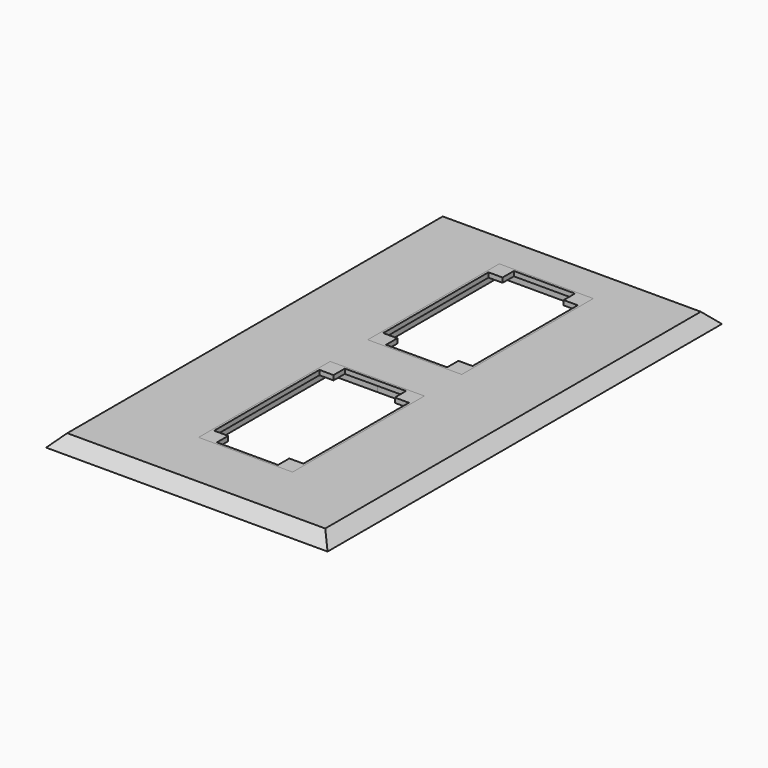
from build123d import *

# Parameters (mm, degrees)
F0_W        = 120
F0_H        = 210
F1_DEPTH    = 5
F2_DEPTH    = 2
F3_T1_DEPTH = 236.1282991577
F3_T3_DEPTH = 146.1282991577


# Not quite as in the source:
# - a fillet or chamfer that OpenCascade refuses, or shapes differently, is made with other operations: its cross-section is extruded or revolved along the edge and cut away or added


with BuildPart() as f1:
    # F0 (on Top) → F1 (new body)
    with BuildSketch(Plane.XY):
        Rectangle(F0_W, F0_H)
        Polygon((20.0805937573, -4.8363452922), (21.0805937573, -4.8321490176), (21.0805937573, -5.8321578219), (21.0805937573, -75), (-18.9194062427, -75), (-18.9194062427, -5), (1.0805937573, -4.9160745088), (14.0805937573, -4.8615229395), align=None, mode=Mode.SUBTRACT)
        Polygon((-18.9194062427, 22), (-18.9194062427, 52.2003881633), (-18.9194062427, 78), (-18.9194062427, 85), (-11.9194062427, 85), (14.0805937573, 85), (21.0805937573, 85), (21.0805937573, 78), (21.0805937573, 50.9695373476), (21.0805937573, 15), (14.0805937573, 15), (-11.9194062427, 15), (-18.9194062427, 15), align=None, mode=Mode.SUBTRACT)
    extrude(amount=-F1_DEPTH)

    # F3: chamfer of 5.08 on 4 edges, made by hand

    # F3_s2 → F3_t1 (cut)
    with BuildSketch(Plane.XZ.offset(-118.0641495789)):
        Polygon((-54.92, 0), (-60, -5.08), (-60, 0), align=None)
        Polygon((54.92, 0), (60, -5.08), (60, 0), align=None)
    extrude(amount=F3_T1_DEPTH, mode=Mode.SUBTRACT)

    # F3_s4 → F3_t3 (cut)
    with BuildSketch(Plane.YZ.offset(-73.0641495789)):
        Polygon((105, -5.08), (99.92, 0), (105, 0), align=None)
        Polygon((-105, -5.08), (-99.92, 0), (-105, 0), align=None)
    extrude(amount=F3_T3_DEPTH, mode=Mode.SUBTRACT)


with BuildPart() as f2:
    # F0 (on Top) → F2 (new body)
    with BuildSketch(Plane.XY):
        Polygon((21.0805937573, -5.8321578219), (21.0805937573, -4.8321490176), (20.0805937573, -4.8363452922), (14.0805937573, -4.8615229395), (1.0805937573, -4.9160745088), (-18.9194062427, -5), (-18.9194062427, -75), (21.0805937573, -75), align=None)
        Polygon((14.0554163316, -5.8616373952), (14.0805937573, -11.8615845698), (20.0805937573, -11.8615845698), (20.0805937573, -68), (14.0805937573, -68), (14.0805937573, -74), (-11.9194062427, -74), (-11.9194062427, -68), (-17.9194062427, -68), (-17.9194062427, -11.9706877083), (-11.9194062427, -11.9706877083), (-11.9194062427, -5.9706348824), align=None, mode=Mode.SUBTRACT)
    extrude(amount=-F2_DEPTH)


with BuildPart() as f2b:
    # F0 (on Top) → F2, piece 2 (new body)
    with BuildSketch(Plane.XY):
        Polygon((-18.9194062427, 78), (-18.9194062427, 52.2003881633), (-18.9194062427, 22), (-18.9194062427, 15), (-11.9194062427, 15), (14.0805937573, 15), (21.0805937573, 15), (21.0805937573, 50.9695373476), (21.0805937573, 78), (21.0805937573, 85), (14.0805937573, 85), (-11.9194062427, 85), (-18.9194062427, 85), align=None)
        Polygon((-17.9194062427, 22), (-17.9194062427, 78), (-11.9194062427, 78), (-11.9194062427, 84), (14.0805937573, 84), (14.0805937573, 78), (20.0805937573, 78), (20.0805937573, 22), (14.0805937573, 22), (14.0805937573, 16), (-11.9194062427, 16), (-11.9194062427, 22), align=None, mode=Mode.SUBTRACT)
    extrude(amount=-F2_DEPTH)


solid = Compound([f1.part, f2.part, f2b.part])
